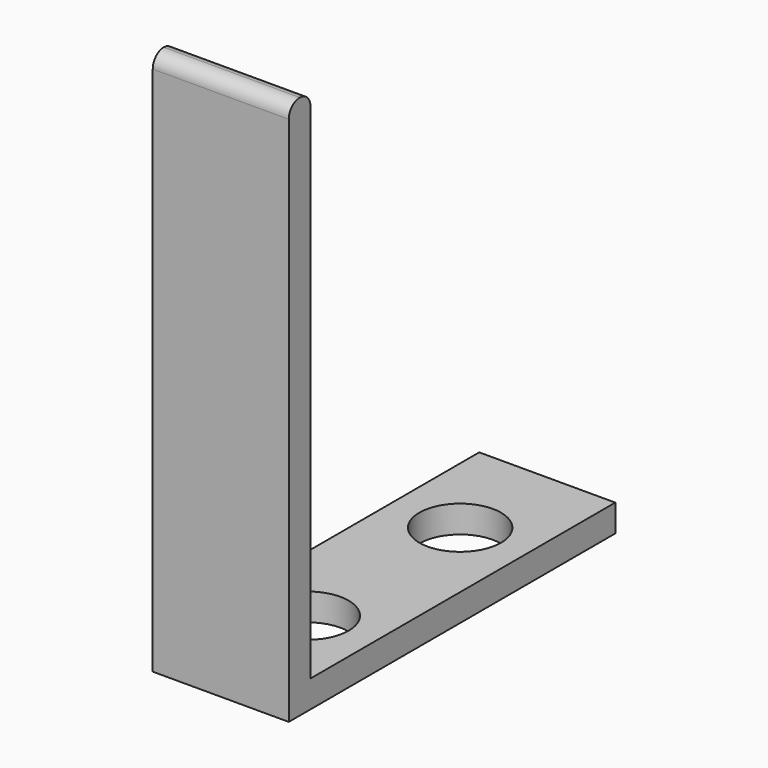
from build123d import *

# Parameters (mm, degrees)
F1_DEPTH = 2.5
F2_R     = 1.5
F3_DEPTH = 1
F4_R     = 0.49999


# Not quite as in the source:
# - a fillet or chamfer is up to 0.001 mm smaller than in the source, because OpenCascade refuses the exact size


with BuildPart() as f1:
    # F0 (on Right) → F1 (new body, symmetric)
    with BuildSketch(Plane.YZ):
        Polygon((-7.5, 0), (7.5, 0), (7.5, 1), (-6.5, 1), (-6.5, 20), (-7.5, 20), align=None)
    extrude(amount=F1_DEPTH, both=True)

    # F2 (on face) → F3 (cut, through all)
    with BuildSketch(Plane.XY.offset(1)):
        with Locations((0, 3.5)):
            Circle(F2_R)
        with Locations((0, -3.5)):
            Circle(F2_R)
    extrude(amount=-F3_DEPTH, mode=Mode.SUBTRACT)

    # F4 (radius 0.5 in the source; OpenCascade refuses exactly that, so slightly less here)
    f4_edges = [f1.edges().sort_by_distance(p)[0] for p in [
        (0, -6.5, 20),
        (0, -7.5, 20),
    ]]
    fillet(f4_edges, radius=F4_R)


solid = f1.part
